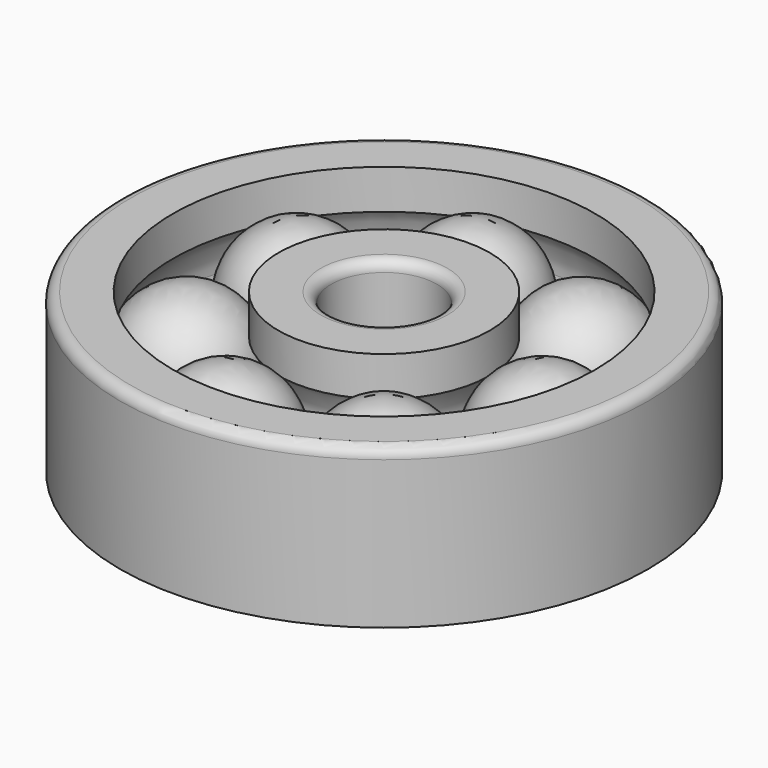
from build123d import *

# Parameters (mm, degrees)
F4_COPIES_COUNT = 7
F5_R            = 2.54
F5_2_R          = 2.54


# Not quite as in the source:
# - a pattern or mirror of a feature is missing from the dataset's text; its kind, count and spacing are read off the source's solid


with BuildPart() as f1:
    # F0 (on Front) → F1 (revolve)
    with BuildSketch(Plane.XZ):
        with BuildLine():
            Line((50.8, 19.05), (50.8, 9.525))
            ThreePointArc((50.8, 9.525), (53.1603473566, 5.0201157855), (53.975, 0))
            ThreePointArc((53.975, 0), (53.1603473566, -5.0201157855), (50.8, -9.525))
            Line((50.8, -9.525), (50.8, -19.05))
            Line((50.8, -19.05), (63.5, -19.05))
            Line((63.5, -19.05), (63.5, 19.05))
            Line((63.5, 19.05), (50.8, 19.05))
        make_face()
    revolve(axis=Axis((0, 0, 0), (0, 0, -1)))

    # F5
    f5_edges = [f1.edges().sort_by_distance(p)[0] for p in [
        (-63.5, 0, 19.05),
    ]]
    fillet(f5_edges, radius=F5_R)


with BuildPart() as f1b:
    # F0 (on Front) → F1, piece 2 (revolve)
    with BuildSketch(Plane.XZ):
        with BuildLine():
            Line((25.4, 19.05), (12.7, 19.05))
            Line((12.7, 19.05), (12.7, -19.05))
            Line((12.7, -19.05), (25.4, -19.05))
            Line((25.4, -19.05), (25.4, -9.525))
            ThreePointArc((25.4, -9.525), (23.0396526434, -5.0201157855), (22.225, 0))
            ThreePointArc((22.225, 0), (23.0396526434, 5.0201157855), (25.4, 9.525))
            Line((25.4, 9.525), (25.4, 19.05))
        make_face()
    revolve(axis=Axis((0, 0, 0), (0, 0, -1)))

    # F5#2
    f5_2_edges = [f1b.edges().sort_by_distance(p)[0] for p in [
        (-12.7, 0, 19.05),
    ]]
    fillet(f5_2_edges, radius=F5_2_R)


with BuildPart() as f4:
    # F3 (on face) → F4 (revolve)
    with BuildSketch(Plane.XZ):
        with BuildLine():
            Line((50.8, 0), (53.975, 0))
            ThreePointArc((53.975, 0), (38.1, 15.875), (22.225, 0))
            Line((22.225, 0), (25.4, 0))
            Line((25.4, 0), (50.8, 0))
        make_face()
    revolve(axis=Axis((38.1, 0, 0), (1, 0, 0)))


with BuildPart() as f4_copies_1:
    # F4_copies: instance of F4
    add(f4.part.rotate(Axis((0, 0, 0), (0, 0, 1)), 1 * 360 / F4_COPIES_COUNT))


with BuildPart() as f4_copies_2:
    # F4_copies: instance of F4
    add(f4.part.rotate(Axis((0, 0, 0), (0, 0, 1)), 2 * 360 / F4_COPIES_COUNT))


with BuildPart() as f4_copies_3:
    # F4_copies: instance of F4
    add(f4.part.rotate(Axis((0, 0, 0), (0, 0, 1)), 3 * 360 / F4_COPIES_COUNT))


with BuildPart() as f4_copies_4:
    # F4_copies: instance of F4
    add(f4.part.rotate(Axis((0, 0, 0), (0, 0, 1)), 4 * 360 / F4_COPIES_COUNT))


with BuildPart() as f4_copies_5:
    # F4_copies: instance of F4
    add(f4.part.rotate(Axis((0, 0, 0), (0, 0, 1)), 5 * 360 / F4_COPIES_COUNT))


with BuildPart() as f4_copies_6:
    # F4_copies: instance of F4
    add(f4.part.rotate(Axis((0, 0, 0), (0, 0, 1)), 6 * 360 / F4_COPIES_COUNT))


solid = Compound([f1.part, f1b.part, f4.part, f4_copies_1.part, f4_copies_2.part, f4_copies_3.part, f4_copies_4.part, f4_copies_5.part, f4_copies_6.part])
